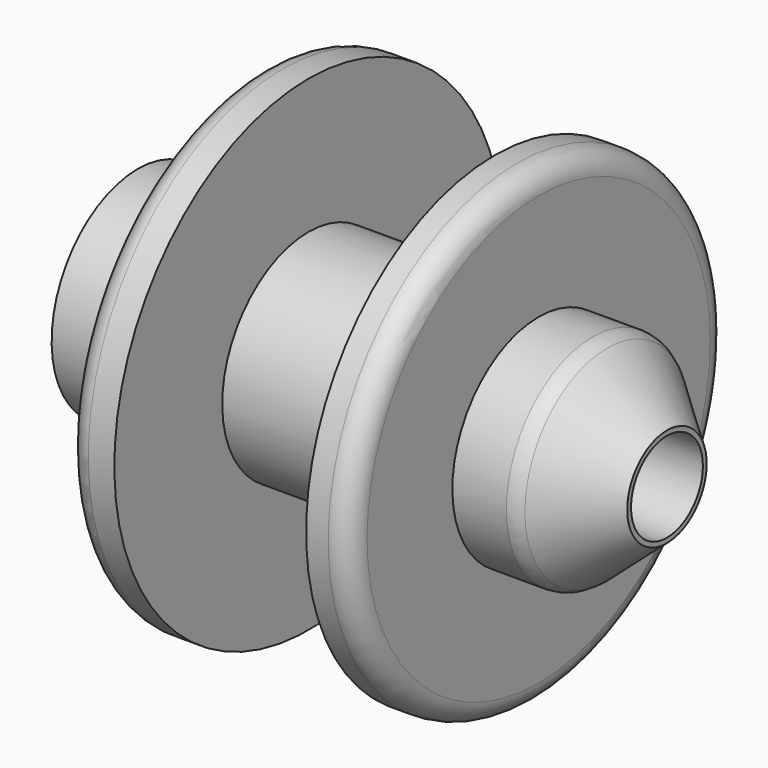
from build123d import *

# Parameters (mm, degrees)
F2_R     = 10.5676667099
F3_DEPTH = 124.5231421123
F4_R     = 5.08


# Not quite as in the source:
# - a feature names something its author has since deleted; it is built from what else it names


with BuildPart() as f1:
    # F0 (on Front) → F1 (revolve)
    with BuildSketch(Plane.XZ):
        Polygon((0, 25.3843758255), (0, 0), (124.5221421123, 0), (124.5221421123, 11.6869108751), (108.956836164, 25.3843758255), (94.325453043, 25.3843758255), (94.325453043, 55.5810630322), (84.0523540974, 55.5810630322), (84.0523540974, 25.3843758255), (40.1582047343, 25.3843758255), (40.1582047343, 57.137593627), (28.951190412, 57.137593627), (28.951190412, 25.3843758255), align=None)
    revolve(axis=Axis((62.2610710561, 0, 0), (1, 0, 0)))

    # F2 (on Right) → F3 (cut, through all)
    with BuildSketch(Plane.YZ):
        Circle(F2_R)
    extrude(amount=F3_DEPTH, mode=Mode.SUBTRACT)

    # F4
    f4_edges = [f1.edges().sort_by_distance(p)[0] for p in [
        (108.956836, 0, -25.384376),
        (94.325453, 0, -55.581063),
        (28.95119, 0, -57.137594),
    ]]
    fillet(f4_edges, radius=F4_R)


solid = f1.part
